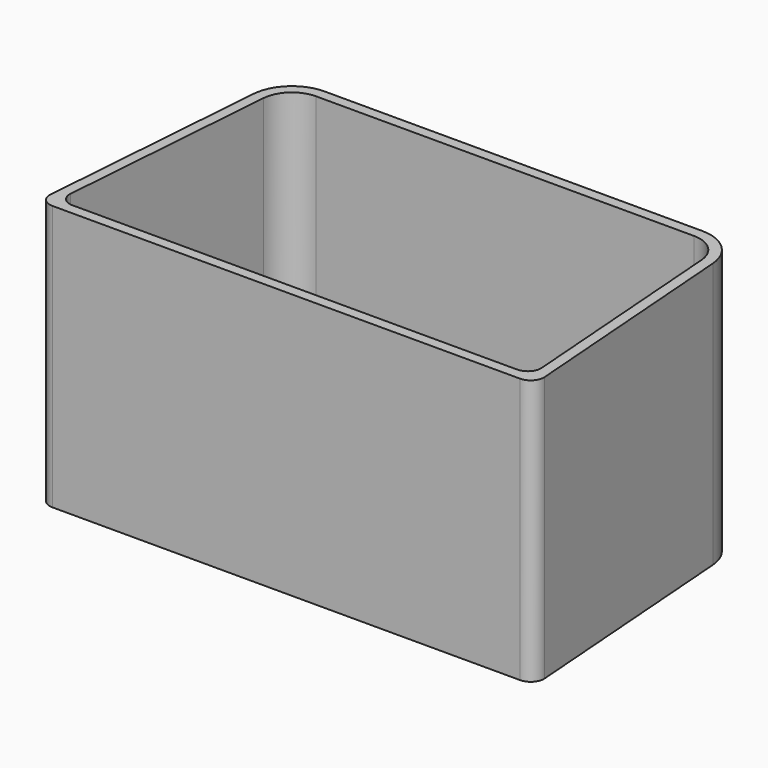
from build123d import *

# Parameters (mm, degrees)
F1_DEPTH = 100
F2_T     = -4
F3_R     = 5


with BuildPart() as f1:
    # F0 (on Top) → F1 (new body)
    with BuildSketch(Plane.XY):
        with BuildLine():
            Line((-74.9023482991, 51.9376612258), (-81.8753698939, -40.8005561921))
            Line((-81.8753698939, -40.8005561921), (105.1246301061, -40.8005561921))
            Line((105.1246301061, -40.8005561921), (98.1516085112, 51.9376612258))
            ThreePointArc((98.1516085112, 51.9376612258), (93.2625692956, 62.0850012182), (82.7772187745, 66.1994438079))
            Line((82.7772187745, 66.1994438079), (-59.5279585624, 66.1994438079))
            ThreePointArc((-59.5279585624, 66.1994438079), (-70.0133090834, 62.0850012182), (-74.9023482991, 51.9376612258))
        make_face()
    extrude(amount=F1_DEPTH)

    # F2
    f2_openings = [f1.faces().sort_by_distance(p)[0] for p in [
        (11.62463, 11.668388, 100),
    ]]
    offset(amount=F2_T, openings=f2_openings)

    # F3
    f3_edges = [f1.edges().sort_by_distance(p)[0] for p in [
        (105.12463, -40.800556, 50),
        (-81.87537, -40.800556, 50),
        (100.812577, -36.800556, 52),
        (-77.563317, -36.800556, 52),
        (11.62463, -36.800556, 4),
        (97.487723, 7.418595, 4),
    ]]
    fillet(f3_edges, radius=F3_R)


solid = f1.part
